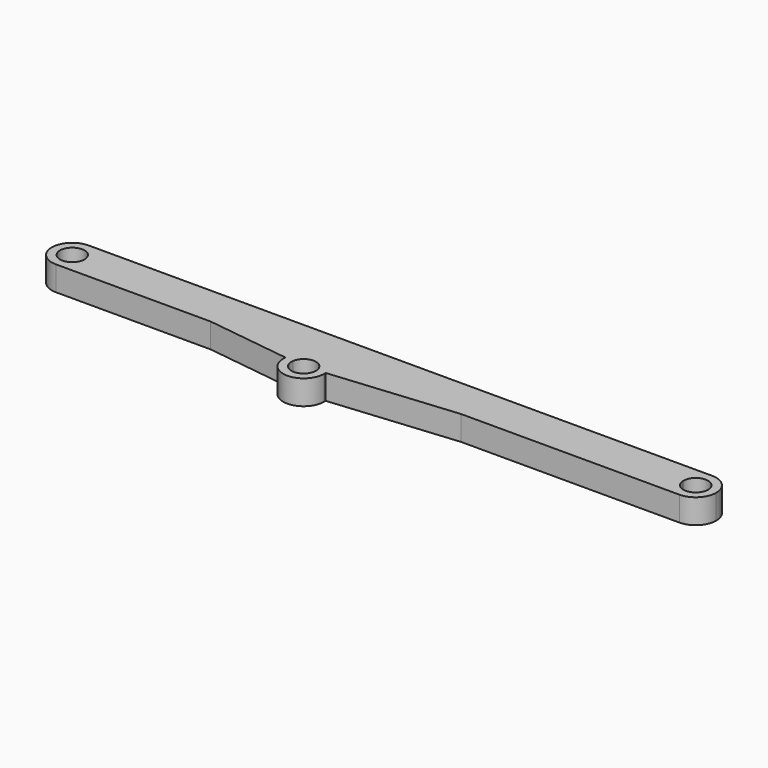
from build123d import *

# Parameters (mm, degrees)
F1_DEPTH = 3


# Not quite as in the source:
# - a feature of the source that left no trace in its solid (it failed there, or was rolled back) is left out


with BuildPart() as f1:
    # F0 (on Top) → F1 (new body)
    with BuildSketch(Plane.XY):
        with BuildLine():
            ThreePointArc((-20.1571040975, 8.6286983024), (-18.3893371446, 7.8964652554), (-17.6571040975, 6.1286983024))
            Line((-17.6571040975, 6.1286983024), (53.465291932, 6.1286983024))
            ThreePointArc((53.465291932, 6.1286983024), (54.1975249791, 7.8964652554), (55.965291932, 8.6286983024))
            Line((55.965291932, 8.6286983024), (-20.1571040975, 8.6286983024))
        make_face()
        with BuildLine():
            Line((-18.6571040975, 6.1286983024), (-17.6571040975, 6.1286983024))
            ThreePointArc((-17.6571040975, 6.1286983024), (-18.3893371446, 7.8964652554), (-20.1571040975, 8.6286983024))
            ThreePointArc((-20.1571040975, 8.6286983024), (-22.6571040975, 6.1286983024), (-20.1571040975, 3.6286983024))
            ThreePointArc((-20.1571040975, 3.6286983024), (-18.5092794047, 4.2486254895), (-17.6786797732, 5.800959277))
            Line((-17.6786797732, 5.800959277), (-18.670049503, 5.9320548872))
            ThreePointArc((-18.670049503, 5.9320548872), (-21.6538642473, 6.2272328348), (-18.6571040975, 6.1286983024))
        make_face()
        with BuildLine():
            Line((53.465291932, 6.1286983024), (-17.6571040975, 6.1286983024))
            ThreePointArc((-17.6571040975, 6.1286983024), (-17.6625038479, 5.9644740818), (-17.6786797732, 5.800959277))
            Line((-17.6786797732, 5.800959277), (-1.2516325751, 3.6286983024))
            Line((-1.2516325751, 3.6286983024), (9.58356384, 3.6286983024))
            ThreePointArc((9.58356384, 3.6286983024), (11.4368578188, 4.4508123027), (13.2901517977, 3.6286983024))
            Line((13.2901517977, 3.6286983024), (29.319977701, 3.6286983024))
            Line((29.319977701, 3.6286983024), (53.476223752, 5.8951611635))
            ThreePointArc((53.476223752, 5.8951611635), (53.4680263825, 6.011801874), (53.465291932, 6.1286983024))
        make_face()
        with BuildLine():
            ThreePointArc((55.965291932, 8.6286983024), (54.1975249791, 7.8964652554), (53.465291932, 6.1286983024))
            Line((53.465291932, 6.1286983024), (54.465291932, 6.1286983024))
            ThreePointArc((54.465291932, 6.1286983024), (55.965291932, 7.6286983024), (57.465291932, 6.1286983024))
            ThreePointArc((57.465291932, 6.1286983024), (56.0354297891, 4.6303389727), (54.471851024, 5.9885760191))
            Line((54.471851024, 5.9885760191), (53.476223752, 5.8951611635))
            ThreePointArc((53.476223752, 5.8951611635), (54.2821167848, 4.2802066406), (55.965291932, 3.6286983024))
            ThreePointArc((55.965291932, 3.6286983024), (57.733058885, 4.3609313494), (58.465291932, 6.1286983024))
            ThreePointArc((58.465291932, 6.1286983024), (57.733058885, 7.8964652554), (55.965291932, 8.6286983024))
        make_face()
        with BuildLine():
            Line((-1.2516325751, 3.6286983024), (-17.6786797732, 5.800959277))
            ThreePointArc((-17.6786797732, 5.800959277), (-18.5092794047, 4.2486254895), (-20.1571040975, 3.6286983024))
            Line((-20.1571040975, 3.6286983024), (-1.2516325751, 3.6286983024))
        make_face()
        with BuildLine():
            ThreePointArc((55.965291932, 3.6286983024), (54.2821167848, 4.2802066406), (53.476223752, 5.8951611635))
            Line((53.476223752, 5.8951611635), (29.319977701, 3.6286983024))
            Line((29.319977701, 3.6286983024), (55.965291932, 3.6286983024))
        make_face()
        with BuildLine():
            Line((9.58356384, 3.6286983024), (-1.2516325751, 3.6286983024))
            Line((-1.2516325751, 3.6286983024), (8.9584334945, 2.2785513281))
            ThreePointArc((8.9584334945, 2.2785513281), (9.1682304635, 3.0012074295), (9.58356384, 3.6286983024))
        make_face()
        with BuildLine():
            Line((13.9259259989, 2.1843494416), (29.319977701, 3.6286983024))
            Line((29.319977701, 3.6286983024), (13.2901517977, 3.6286983024))
            ThreePointArc((13.2901517977, 3.6286983024), (13.7249931268, 2.9580048426), (13.9259259989, 2.1843494416))
        make_face()
        with BuildLine():
            ThreePointArc((9.58356384, 3.6286983024), (9.1682304635, 3.0012074295), (8.9584334945, 2.2785513281))
            Line((8.9584334945, 2.2785513281), (9.9498032243, 2.1474557179))
            ThreePointArc((9.9498032243, 2.1474557179), (11.4652982098, 3.4505426599), (12.9302987268, 2.090934586))
            Line((12.9302987268, 2.090934586), (13.9259259989, 2.1843494416))
            ThreePointArc((13.9259259989, 2.1843494416), (13.7249931268, 2.9580048426), (13.2901517977, 3.6286983024))
            Line((13.2901517977, 3.6286983024), (9.58356384, 3.6286983024))
        make_face()
        with BuildLine():
            Line((9.9498032243, 2.1474557179), (8.9584334945, 2.2785513281))
            ThreePointArc((8.9584334945, 2.2785513281), (11.2726335982, -0.5437879469), (13.9368578188, 1.9508123027))
            ThreePointArc((13.9368578188, 1.9508123027), (13.9341233684, 2.0677087311), (13.9259259989, 2.1843494416))
            Line((13.9259259989, 2.1843494416), (12.9302987268, 2.090934586))
            ThreePointArc((12.9302987268, 2.090934586), (12.9352171486, 2.0209501598), (12.9368578188, 1.9508123027))
            ThreePointArc((12.9368578188, 1.9508123027), (11.3383232865, 0.4540521529), (9.9498032243, 2.1474557179))
        make_face()
        with BuildLine():
            ThreePointArc((13.2901517977, 3.6286983024), (11.4368578188, 4.4508123027), (9.58356384, 3.6286983024))
            Line((9.58356384, 3.6286983024), (13.2901517977, 3.6286983024))
        make_face()
        with BuildLine():
            ThreePointArc((-17.6786797732, 5.800959277), (-17.6625038479, 5.9644740818), (-17.6571040975, 6.1286983024))
            Line((-17.6571040975, 6.1286983024), (-18.6571040975, 6.1286983024))
            ThreePointArc((-18.6571040975, 6.1286983024), (-18.6603439478, 6.03016377), (-18.670049503, 5.9320548872))
            Line((-18.670049503, 5.9320548872), (-17.6786797732, 5.800959277))
        make_face()
        with BuildLine():
            Line((54.465291932, 6.1286983024), (53.465291932, 6.1286983024))
            ThreePointArc((53.465291932, 6.1286983024), (53.4680263825, 6.011801874), (53.476223752, 5.8951611635))
            Line((53.476223752, 5.8951611635), (54.471851024, 5.9885760191))
            ThreePointArc((54.471851024, 5.9885760191), (54.4669326023, 6.0585604453), (54.465291932, 6.1286983024))
        make_face()
    extrude(amount=F1_DEPTH)


solid = f1.part
